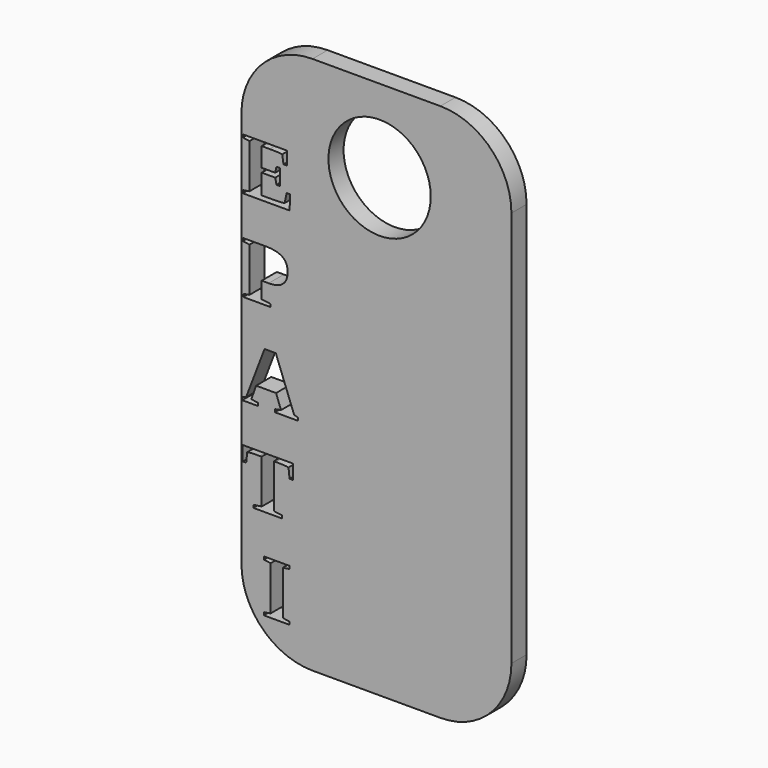
from build123d import *

# Parameters (mm, degrees)
F0_R     = 27.432
F1_DEPTH = 10.16


with BuildPart() as f1:
    # F0 (on Front) → F1 (new body)
    with BuildSketch(Plane.XZ):
        with BuildLine():
            ThreePointArc((0, -38.4786100226), (11.1592316368, -65.4193783858), (38.1, -76.5786100226))
            Line((38.1, -76.5786100226), (106.68, -76.5786100226))
            ThreePointArc((106.68, -76.5786100226), (133.6207683632, -65.4193783858), (144.78, -38.4786100226))
            Line((144.78, -38.4786100226), (144.78, 174.1193899774))
            ThreePointArc((144.78, 174.1193899774), (133.6207683632, 201.0601583406), (106.68, 212.2193899774))
            Line((106.68, 212.2193899774), (38.1, 212.2193899774))
            ThreePointArc((38.1, 212.2193899774), (11.1592316368, 201.0601583406), (0, 174.1193899774))
            Line((0, 174.1193899774), (0, -38.4786100226))
        make_face()
        Polygon((22.1777712578, -33.1991309873), (22.1777712578, -56.8850969951), (25.7456152258, -57.4299074334), (25.7456152258, -58.9646783023), (12.065558, -58.9646783023), (12.065558, -57.4299074334), (15.6334019681, -56.8850969951), (15.6334019681, -33.1991309873), (12.065558, -32.6343884598), (12.065558, -31.11954968), (25.7456152258, -31.11954968), (25.7456152258, -32.6343884598), align=None, mode=Mode.SUBTRACT)
        with BuildLine():
            Line((21.845569771, -10.0646194476), (6.4380648139, -10.0646194476))
            Line((6.4380648139, -10.0646194476), (6.4380648139, -8.5497806678))
            Line((6.4380648139, -8.5497806678), (10.8563445881, -7.9850381403))
            Line((10.8563445881, -7.9850381403), (10.8563445881, 15.5746913025))
            Line((10.8563445881, 15.5746913025), (9.7999438602, 15.5746913025))
            add(Edge.make_bspline(
                [(9.7999438602, 15.5746913025), (5.0428185694, 15.5746913025), (3.116049946, 15.1627614589)],
                knots=[0, 0, 0, 1, 1, 1], degree=2))
            Line((3.116049946, 15.1627614589), (2.5513074185, 9.9937063245))
            Line((2.5513074185, 9.9937063245), (0.6644029736, 9.9937063245))
            Line((0.6644029736, 9.9937063245), (0.6644029736, 17.7805091747))
            Line((0.6644029736, 17.7805091747), (27.7188920573, 17.7805091747))
            Line((27.7188920573, 17.7805091747), (27.7188920573, 9.9937063245))
            Line((27.7188920573, 9.9937063245), (25.8054114935, 9.9937063245))
            Line((25.8054114935, 9.9937063245), (25.2473129957, 15.1627614589))
            add(Edge.make_bspline(
                [(25.2473129957, 15.1627614589), (23.5265092941, 15.5348271241), (18.4371825166, 15.5348271241)],
                knots=[0, 0, 0, 1, 1, 1], degree=2))
            Line((18.4371825166, 15.5348271241), (17.420645967, 15.5348271241))
            Line((17.420645967, 15.5348271241), (17.420645967, -7.9850381403))
            Line((17.420645967, -7.9850381403), (21.845569771, -8.5497806678))
            Line((21.845569771, -8.5497806678), (21.845569771, -10.0646194476))
        make_face(mode=Mode.SUBTRACT)
        Polygon((5.3152237886, 40.9150207144), (8.8897117864, 40.3502781869), (8.8897117864, 38.8354394072), (0.4185738733, 38.8354394072), (0.4185738733, 40.3502781869), (2.4915111509, 40.9150207144), (12.3977594868, 66.9064650405), (18.4172504274, 66.9064650405), (28.2769905551, 40.9150207144), (30.3964360408, 40.3502781869), (30.3964360408, 38.8354394072), (17.998676554, 38.8354394072), (17.998676554, 40.3502781869), (21.2210309758, 40.9150207144), (18.5634190815, 48.1171489479), (7.8665312071, 48.1171489479), align=None, mode=Mode.SUBTRACT)
        with BuildLine():
            Line((14.5969333293, 98.6582831474), (10.8563445881, 98.6582831474))
            Line((10.8563445881, 98.6582831474), (10.8563445881, 89.8150795692))
            Line((10.8563445881, 89.8150795692), (15.4872333139, 89.2503370416))
            Line((15.4872333139, 89.2503370416), (15.4872333139, 87.7354982619))
            Line((15.4872333139, 87.7354982619), (0.9966044604, 87.7354982619))
            Line((0.9966044604, 87.7354982619), (0.9966044604, 89.2503370416))
            Line((0.9966044604, 89.2503370416), (4.298687239, 89.8150795692))
            Line((4.298687239, 89.8150795692), (4.298687239, 113.5209776661))
            Line((4.298687239, 113.5209776661), (0.7241992412, 114.0657881045))
            Line((0.7241992412, 114.0657881045), (0.7241992412, 115.5806268842))
            Line((0.7241992412, 115.5806268842), (12.995722163, 115.5806268842))
            add(Edge.make_bspline(
                [(12.995722163, 115.5806268842), (18.9155526575, 115.5806268842), (21.8422477561, 113.5973840081)],
                knots=[0, 0, 0, 1, 1, 1], degree=2))
            add(Edge.make_bspline(
                [(21.8422477561, 113.5973840081), (24.7689428547, 111.614141132), (24.7689428547, 107.3752501606)],
                knots=[0, 0, 0, 1, 1, 1], degree=2))
            add(Edge.make_bspline(
                [(24.7689428547, 107.3752501606), (24.7689428547, 98.6582831474), (14.5969333293, 98.6582831474)],
                knots=[0, 0, 0, 1, 1, 1], degree=2))
        make_face(mode=Mode.SUBTRACT)
        with BuildLine():
            Line((0.7241992412, 136.6355571166), (0.7241992412, 138.1503958964))
            Line((0.7241992412, 138.1503958964), (4.298687239, 138.7151384239))
            Line((4.298687239, 138.7151384239), (4.298687239, 162.4210365209))
            Line((4.298687239, 162.4210365209), (0.7241992412, 162.9658469592))
            Line((0.7241992412, 162.9658469592), (0.7241992412, 164.4806857389))
            Line((0.7241992412, 164.4806857389), (24.4367413679, 164.4806857389))
            Line((24.4367413679, 164.4806857389), (24.4367413679, 157.3981500407))
            Line((24.4367413679, 157.3981500407), (22.549836923, 157.3981500407))
            Line((22.549836923, 157.3981500407), (21.8854339494, 161.9028022015))
            add(Edge.make_bspline(
                [(21.8854339494, 161.9028022015), (19.5600235419, 162.1951395099), (15.1550318271, 162.1951395099)],
                knots=[0, 0, 0, 1, 1, 1], degree=2))
            Line((15.1550318271, 162.1951395099), (10.8364124989, 162.1951395099))
            Line((10.8364124989, 162.1951395099), (10.8364124989, 151.9766217764))
            Line((10.8364124989, 151.9766217764), (18.124913119, 151.9766217764))
            Line((18.124913119, 151.9766217764), (18.7693840033, 155.052807544))
            Line((18.7693840033, 155.052807544), (20.6164242699, 155.052807544))
            Line((20.6164242699, 155.052807544), (20.6164242699, 146.4952972444))
            Line((20.6164242699, 146.4952972444), (18.7693840033, 146.4952972444))
            Line((18.7693840033, 146.4952972444), (18.124913119, 149.6512113689))
            Line((18.124913119, 149.6512113689), (10.8364124989, 149.6512113689))
            Line((10.8364124989, 149.6512113689), (10.8364124989, 138.9211033457))
            Line((10.8364124989, 138.9211033457), (16.0918400199, 138.9211033457))
            add(Edge.make_bspline(
                [(16.0918400199, 138.9211033457), (21.4469279868, 138.9211033457), (23.1079354208, 139.2533048325)],
                knots=[0, 0, 0, 1, 1, 1], degree=2))
            Line((23.1079354208, 139.2533048325), (24.2905727137, 144.4024278777))
            Line((24.2905727137, 144.4024278777), (26.1841211884, 144.4024278777))
            Line((26.1841211884, 144.4024278777), (25.7854794042, 136.6355571166))
            Line((25.7854794042, 136.6355571166), (0.7241992412, 136.6355571166))
        make_face(mode=Mode.SUBTRACT)
        with Locations((74.0844953617, 167.8276180772)):
            Circle(F0_R, mode=Mode.SUBTRACT)
    extrude(amount=F1_DEPTH)


solid = f1.part
